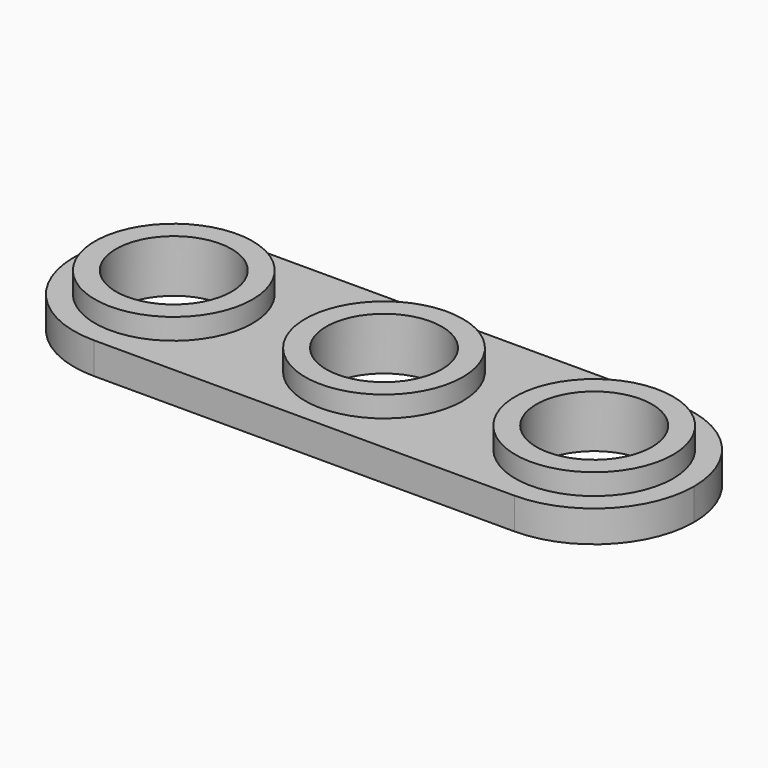
from build123d import *

# Parameters (mm, degrees)
F2_R     = 7.5
F2_R_2   = 5.5
F3_DEPTH = 3
F4_DEPTH = 5


# Not quite as in the source:
# - a feature names something its author has since deleted; it is built from what else it names


with BuildPart() as f3:
    # F2 (on Top) → F3 (new body)
    with BuildSketch(Plane.XY):
        with BuildLine():
            Line((40, 9.5), (0, 9.5))
            ThreePointArc((0, 9.5), (-6.7175144213, 6.7175144213), (-9.5, 0))
            ThreePointArc((-9.5, 0), (-6.7175144213, -6.7175144213), (0, -9.5))
            Line((0, -9.5), (40, -9.5))
            ThreePointArc((40, -9.5), (46.7175144213, -6.7175144213), (49.5, 0))
            ThreePointArc((49.5, 0), (46.7175144213, 6.7175144213), (40, 9.5))
        make_face()
        Circle(F2_R, mode=Mode.SUBTRACT)
        with Locations((20, 0)):
            Circle(F2_R, mode=Mode.SUBTRACT)
        with Locations((40, 0)):
            Circle(F2_R, mode=Mode.SUBTRACT)
        Circle(F2_R)
        Circle(F2_R_2, mode=Mode.SUBTRACT)
    extrude(amount=F3_DEPTH)

    # F2 (on Top) → F4 (join)
    with BuildSketch(Plane.XY):
        Circle(F2_R)
        Circle(F2_R_2, mode=Mode.SUBTRACT)
        with Locations((20, 0)):
            Circle(F2_R)
        with Locations((20, 0)):
            Circle(F2_R_2, mode=Mode.SUBTRACT)
        with Locations((40, 0)):
            Circle(F2_R)
        with Locations((40, 0)):
            Circle(F2_R_2, mode=Mode.SUBTRACT)
    extrude(amount=F4_DEPTH)


solid = f3.part
